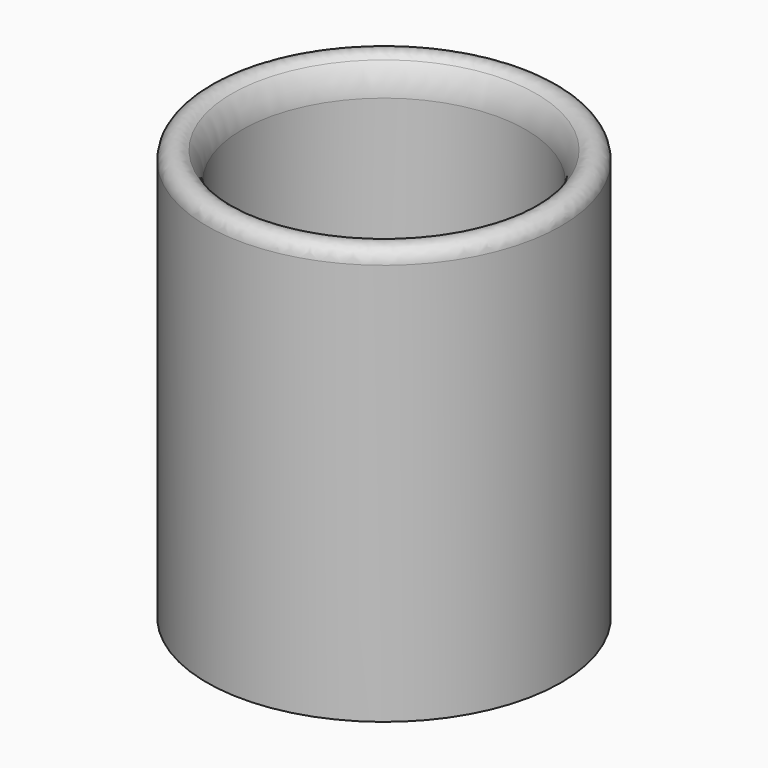
from build123d import *

# Parameters (mm, degrees)
F0_R     = 10
F1_DEPTH = 5
F0_R_2   = 12.5
F2_DEPTH = 30
F4_R     = 1


# Not quite as in the source:
# - a fillet or chamfer that OpenCascade refuses, or shapes differently, is made with other operations: its cross-section is extruded or revolved along the edge and cut away or added


with BuildPart() as f1:
    # F0 (on Top) → F1 (new body)
    with BuildSketch(Plane.XY):
        Circle(F0_R)
    extrude(amount=F1_DEPTH)

    # F0 (on Top) → F2 (join)
    with BuildSketch(Plane.XY):
        Circle(F0_R_2)
        Circle(F0_R, mode=Mode.SUBTRACT)
    extrude(amount=F2_DEPTH)

    # F3: fillet of radius 3 on 1 edges, made by hand

    # F3_s1 → F3_t2 (revolve, cut)
    with BuildSketch(Plane.XZ):
        with BuildLine():
            ThreePointArc((12.5, 30), (10.7087121525, 28.9784517816), (10, 27.0419601084))
            Line((10, 27.0419601084), (10, 30))
            Line((10, 30), (12.5, 30))
        make_face()
    revolve(axis=Axis((0, 0, 30), (0, 0, 1)), mode=Mode.SUBTRACT)

    # F4
    f4_edges = [f1.edges().sort_by_distance(p)[0] for p in [
        (-12.5, 0, 30),
    ]]
    fillet(f4_edges, radius=F4_R)


solid = f1.part
